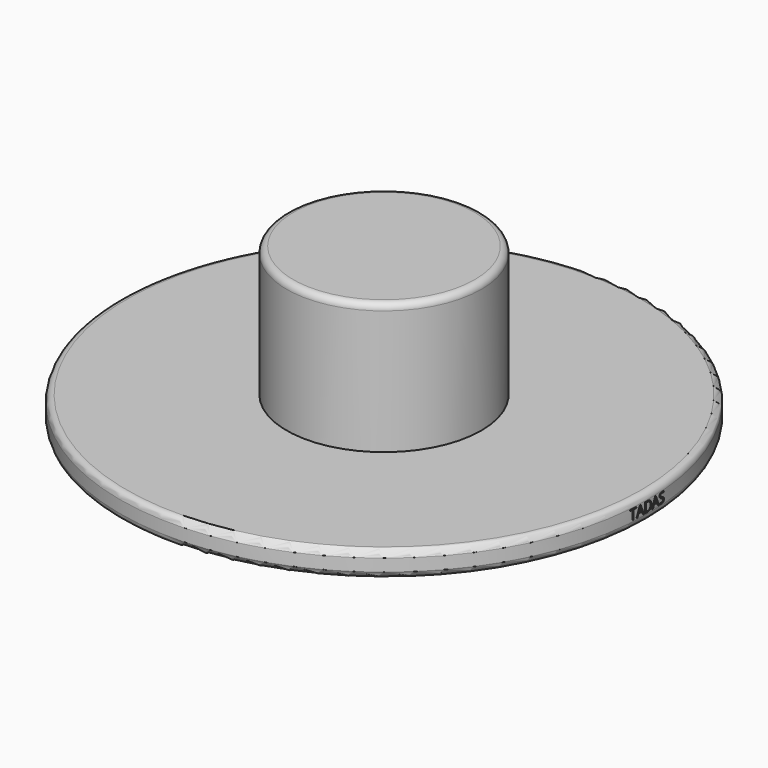
from build123d import *

# Parameters (mm, degrees)
F0_R         = 76.2
F1_DEPTH     = 122.174
F2_T         = -2.54
F0_R_2       = 206.7114105037
F3_DEPTH     = 19.812
F4_R         = 5.08
F6_TEXT_SIZE = 10.950508618
F7_DEPTH     = 71.628


# Not quite as in the source:
# - a feature names something its author has since deleted; it is built from what else it names
# - Text() gives the source's letters only with a copy of the font that has no kerning and outlines rounded to 1/6400 em; it was checked with that copy


with BuildPart() as f1:
    # F0 (on Top) → F1 (new body)
    with BuildSketch(Plane.XY):
        Circle(F0_R)
    extrude(amount=F1_DEPTH)

    # F2
    f2_openings = [f1.faces().sort_by_distance(p)[0] for p in [
        (0, 0, 0),
    ]]
    offset(amount=F2_T, openings=f2_openings)

    # F0 (on Top) → F3 (join)
    with BuildSketch(Plane.XY):
        Circle(F0_R_2)
        Circle(F0_R, mode=Mode.SUBTRACT)
    extrude(amount=F3_DEPTH)

    # F4
    f4_edges = [f1.edges().sort_by_distance(p)[0] for p in [
        (-76.2, 0, 122.174),
        (-206.711411, 0, 19.812),
        (-206.711411, 0, 0),
    ]]
    fillet(f4_edges, radius=F4_R)

    # F6 (on offset) → F7 (cut)
    with BuildSketch(Plane.YZ.offset(208.788)):
        with Locations((-17.0485731047, 6.2716559041)):
            Text('TADAS', F6_TEXT_SIZE, font='Open Sans', text_align=(TextAlign.LEFT, TextAlign.BOTTOM))
    extrude(amount=-F7_DEPTH, mode=Mode.SUBTRACT)


solid = f1.part
